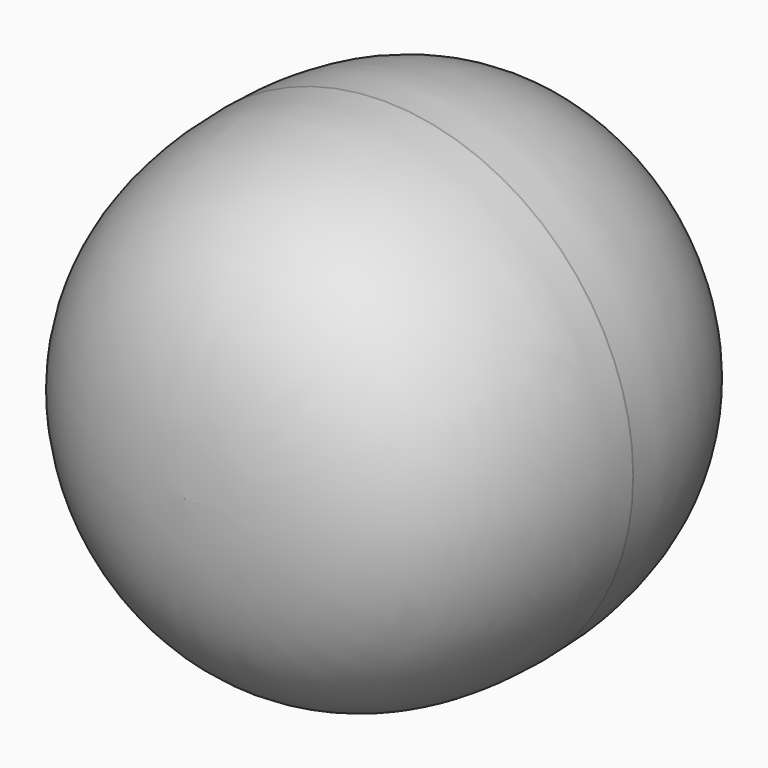
from build123d import *

# Parameters (mm, degrees)
F0_R     = 12.7
F1_DEPTH = 25.4


# Not quite as in the source:
# - a fillet or chamfer that OpenCascade refuses, or shapes differently, is made with other operations: its cross-section is extruded or revolved along the edge and cut away or added


with BuildPart() as f1:
    # F0 (on Front) → F1 (new body)
    with BuildSketch(Plane.XZ):
        Circle(F0_R)
    extrude(amount=F1_DEPTH)

    # F2: fillet of radius 12.6746 on 2 edges, made by hand

    # F2_s1 → F2_t2 (revolve, cut)
    with BuildSketch(Plane.XY):
        with BuildLine():
            add(Edge.make_bspline(
                [(12.7, -12.7254), (12.7, -25.4), (0.0254, -25.4)],
                knots=[0, 0, 0, 1, 1, 1], degree=2, weights=[1, 1, 1]))
            Line((0.0254, -25.4), (12.7, -25.4))
            Line((12.7, -25.4), (12.7, -12.7254))
        make_face()
    revolve(axis=Axis((0, -25.4, 0), (0, -1, 0)), mode=Mode.SUBTRACT)

    # F2_s3 → F2_t4 (revolve, cut)
    with BuildSketch(Plane.XY):
        with BuildLine():
            add(Edge.make_bspline(
                [(12.7, -12.6746), (12.7, 0), (0.0254, 0)],
                knots=[0, 0, 0, 1, 1, 1], degree=2, weights=[1, 1, 1]))
            Line((0.0254, 0), (12.7, 0))
            Line((12.7, 0), (12.7, -12.6746))
        make_face()
    revolve(axis=Axis((0, 0, 0), (0, -1, 0)), mode=Mode.SUBTRACT)


solid = f1.part
